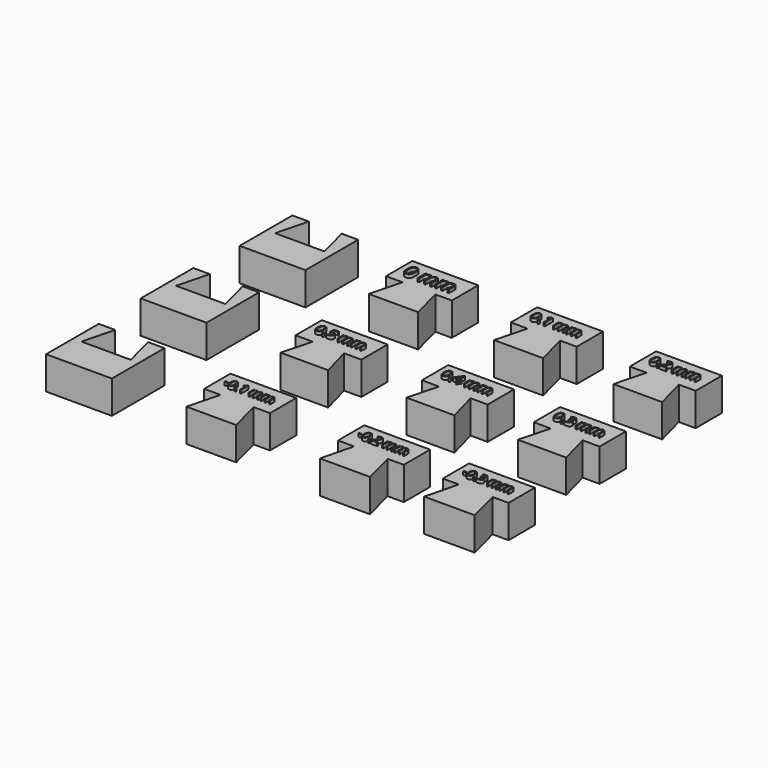
from build123d import *

# Parameters (mm, degrees)
F1_DEPTH      = 10
F2_TEXT_SIZE  = 5.6061667835
F3_DEPTH      = 1
F4_TEXT_SIZE  = 4.2693231344
F5_DEPTH      = 1
F6_TEXT_SIZE  = 4.2693231344
F7_DEPTH      = 1
F8_TEXT_SIZE  = 4.2693231344
F9_DEPTH      = 1
F10_TEXT_SIZE = 4.2693231344
F11_DEPTH     = 1
F12_TEXT_SIZE = 4.2693231344
F13_DEPTH     = 1
F14_TEXT_SIZE = 3.9111835404
F15_DEPTH     = 1
F16_TEXT_SIZE = 3.9111835404
F17_DEPTH     = 1
F18_TEXT_SIZE = 3.9111835404
F19_DEPTH     = 1


# Not quite as in the source:
# - Text() gives the source's letters only with a copy of the font that has no kerning and outlines rounded to 1/6400 em; it was checked with that copy


with BuildPart() as f1:
    # F0 (on Top) → F1 (new body)
    with BuildSketch(Plane.XY):
        Polygon((-54.4452023506, 43.5008010278), (-59.4452023506, 43.5008010278), (-59.4452023506, 23.5008010278), (-39.4452023506, 23.5008010278), (-39.4452023506, 43.5008010278), (-44.4452023506, 43.5008010278), (-41.9452023506, 33.8183426622), (-56.9452023506, 33.8183426622), align=None)
    extrude(amount=F1_DEPTH)


with BuildPart() as f1b:
    # F0 (on Top) → F1, piece 2 (new body)
    with BuildSketch(Plane.XY):
        Polygon((-22.5773579441, 33.0135617405), (-17.5773579441, 33.0135617405), (-20.0773579441, 23.331103375), (-5.0773579441, 23.331103375), (-7.5773579441, 33.0135617405), (-2.5773579441, 33.0135617405), (-2.5773579441, 43.0135617405), (-22.5773579441, 43.0135617405), align=None)
    extrude(amount=F1_DEPTH)

    # F2 (on face) → F3 (join)
    with BuildSketch(Plane.XY.offset(10)):
        with Locations((-20.0773579441, 35.4771216564)):
            Text('0 mm', F2_TEXT_SIZE, font='Open Sans', text_align=(TextAlign.LEFT, TextAlign.BOTTOM))
    extrude(amount=F3_DEPTH)


with BuildPart() as f1c:
    # F0 (on Top) → F1, piece 3 (new body)
    with BuildSketch(Plane.XY):
        Polygon((15.4259026838, 32.9628368528), (20.4759026838, 32.9628368528), (17.9759026838, 23.3836928409), (32.8759026838, 23.3836928409), (30.3759026838, 32.9628368528), (35.4259026838, 32.9628368528), (35.4259026838, 42.9628368528), (15.4259026838, 42.9628368528), align=None)
    extrude(amount=F1_DEPTH)

    # F4 (on face) → F5 (join)
    with BuildSketch(Plane.XY.offset(10)):
        with Locations((17.9259026838, 36.388924196)):
            Text('0.1 mm', F4_TEXT_SIZE, font='Open Sans', text_align=(TextAlign.LEFT, TextAlign.BOTTOM))
    extrude(amount=F5_DEPTH)


with BuildPart() as f1d:
    # F0 (on Top) → F1, piece 4 (new body)
    with BuildSketch(Plane.XY):
        Polygon((51.633169651, 32.8925785896), (56.733169651, 32.8925785896), (54.233169651, 23.4168200448), (69.033169651, 23.4168200448), (66.533169651, 32.8925785896), (71.633169651, 32.8925785896), (71.633169651, 42.8925785896), (51.633169651, 42.8925785896), align=None)
    extrude(amount=F1_DEPTH)

    # F6 (on face) → F7 (join)
    with BuildSketch(Plane.XY.offset(10)):
        with Locations((54.133169651, 36.3186659329)):
            Text('0.2 mm', F6_TEXT_SIZE, font='Open Sans', text_align=(TextAlign.LEFT, TextAlign.BOTTOM))
    extrude(amount=F7_DEPTH)


with BuildPart() as f1e:
    # F0 (on Top) → F1, piece 5 (new body)
    with BuildSketch(Plane.XY):
        Polygon((51.728592962, -3.7110992652), (56.878592962, -3.7110992652), (54.378592962, -13.0833988763), (69.078592962, -13.0833988763), (66.578592962, -3.7110992652), (71.728592962, -3.7110992652), (71.728592962, 6.2889007348), (51.728592962, 6.2889007348), align=None)
    extrude(amount=F1_DEPTH)

    # F12 (on face) → F13 (join)
    with BuildSketch(Plane.XY.offset(10)):
        with Locations((54.228592962, -0.285011922)):
            Text('0.3 mm', F12_TEXT_SIZE, font='Open Sans', text_align=(TextAlign.LEFT, TextAlign.BOTTOM))
    extrude(amount=F13_DEPTH)


with BuildPart() as f1f:
    # F0 (on Top) → F1, piece 6 (new body)
    with BuildSketch(Plane.XY):
        Polygon((17.496650815, -3.4446209112), (22.696650815, -3.4446209112), (20.196650815, -12.7133856616), (34.796650815, -12.7133856616), (32.296650815, -3.4446209112), (37.496650815, -3.4446209112), (37.496650815, 6.5553790888), (17.496650815, 6.5553790888), align=None)
    extrude(amount=F1_DEPTH)

    # F10 (on face) → F11 (join)
    with BuildSketch(Plane.XY.offset(10)):
        with Locations((19.996650815, -0.0185335679)):
            Text('0.4 mm', F10_TEXT_SIZE, font='Open Sans', text_align=(TextAlign.LEFT, TextAlign.BOTTOM))
    extrude(amount=F11_DEPTH)


with BuildPart() as f1g:
    # F0 (on Top) → F1, piece 7 (new body)
    with BuildSketch(Plane.XY):
        Polygon((-20.3525044397, -4.1576060165), (-15.1025044397, -4.1576060165), (-17.6025044397, -13.3227574064), (-3.1025044397, -13.3227574064), (-5.6025044397, -4.1576060165), (-0.3525044397, -4.1576060165), (-0.3525044397, 5.8423939835), (-20.3525044397, 5.8423939835), align=None)
    extrude(amount=F1_DEPTH)

    # F8 (on face) → F9 (join)
    with BuildSketch(Plane.XY.offset(10)):
        with Locations((-17.8525044397, -0.7315186733)):
            Text('0.5 mm', F8_TEXT_SIZE, font='Open Sans', text_align=(TextAlign.LEFT, TextAlign.BOTTOM))
    extrude(amount=F9_DEPTH)


with BuildPart() as f1h:
    # F0 (on Top) → F1, piece 8 (new body)
    with BuildSketch(Plane.XY):
        Polygon((-20.1091777906, -39.1814293651), (-15.1591777906, -39.1814293651), (-17.6591777906, -48.9671332233), (-2.5591777906, -48.9671332233), (-5.0591777906, -39.1814293651), (-0.1091777906, -39.1814293651), (-0.1091777906, -29.1814293651), (-20.1091777906, -29.1814293651), align=None)
    extrude(amount=F1_DEPTH)

    # F14 (on face) → F15 (join)
    with BuildSketch(Plane.XY.offset(10)):
        with Locations((-17.6091777906, -35.6814293651)):
            Text('-0.1 mm', F14_TEXT_SIZE, font='Open Sans', text_align=(TextAlign.LEFT, TextAlign.BOTTOM))
    extrude(amount=F15_DEPTH)


with BuildPart() as f1i:
    # F0 (on Top) → F1, piece 9 (new body)
    with BuildSketch(Plane.XY):
        Polygon((21.2893874943, -40.0706754562), (26.1893874943, -40.0706754562), (23.6893874943, -49.9595581029), (38.8893874943, -49.9595581029), (36.3893874943, -40.0706754562), (41.2893874943, -40.0706754562), (41.2893874943, -30.0706754562), (21.2893874943, -30.0706754562), align=None)
    extrude(amount=F1_DEPTH)

    # F16 (on face) → F17 (join)
    with BuildSketch(Plane.XY.offset(10)):
        with Locations((23.7893874943, -36.5706754562)):
            Text('-0.2 mm', F16_TEXT_SIZE, font='Open Sans', text_align=(TextAlign.LEFT, TextAlign.BOTTOM))
    extrude(amount=F17_DEPTH)


with BuildPart() as f1j:
    # F0 (on Top) → F1, piece 10 (new body)
    with BuildSketch(Plane.XY):
        Polygon((52.945716083, -39.8167642613), (57.795716083, -39.8167642613), (55.295716083, -49.8087610587), (70.595716083, -49.8087610587), (68.095716083, -39.8167642613), (72.945716083, -39.8167642613), (72.945716083, -29.8167642613), (52.945716083, -29.8167642613), align=None)
    extrude(amount=F1_DEPTH)

    # F18 (on face) → F19 (join)
    with BuildSketch(Plane.XY.offset(10)):
        with Locations((55.445716083, -36.3167642613)):
            Text('-0.3 mm', F18_TEXT_SIZE, font='Open Sans', text_align=(TextAlign.LEFT, TextAlign.BOTTOM))
    extrude(amount=F19_DEPTH)


with BuildPart() as f1k:
    # F0 (on Top) → F1, piece 11 (new body)
    with BuildSketch(Plane.XY):
        Polygon((-55.9067960083, 7.7003508308), (-60.9067960083, 7.7003508308), (-60.9067960083, -12.2996491692), (-40.9067960083, -12.2996491692), (-40.9067960083, 7.7003508308), (-45.9067960083, 7.7003508308), (-43.4067960083, -1.9821075347), (-58.4067960083, -1.9821075347), align=None)
    extrude(amount=F1_DEPTH)


with BuildPart() as f1l:
    # F0 (on Top) → F1, piece 12 (new body)
    with BuildSketch(Plane.XY):
        Polygon((-55.5235604942, -28.7321617393), (-60.5235604942, -28.7321617393), (-60.5235604942, -48.7321617393), (-40.5235604942, -48.7321617393), (-40.5235604942, -28.7321617393), (-45.5235604942, -28.7321617393), (-43.0235604942, -38.4146201048), (-58.0235604942, -38.4146201048), align=None)
    extrude(amount=F1_DEPTH)


solid = Compound([f1.part, f1b.part, f1c.part, f1d.part, f1e.part, f1f.part, f1g.part, f1h.part, f1i.part, f1j.part, f1k.part, f1l.part])
